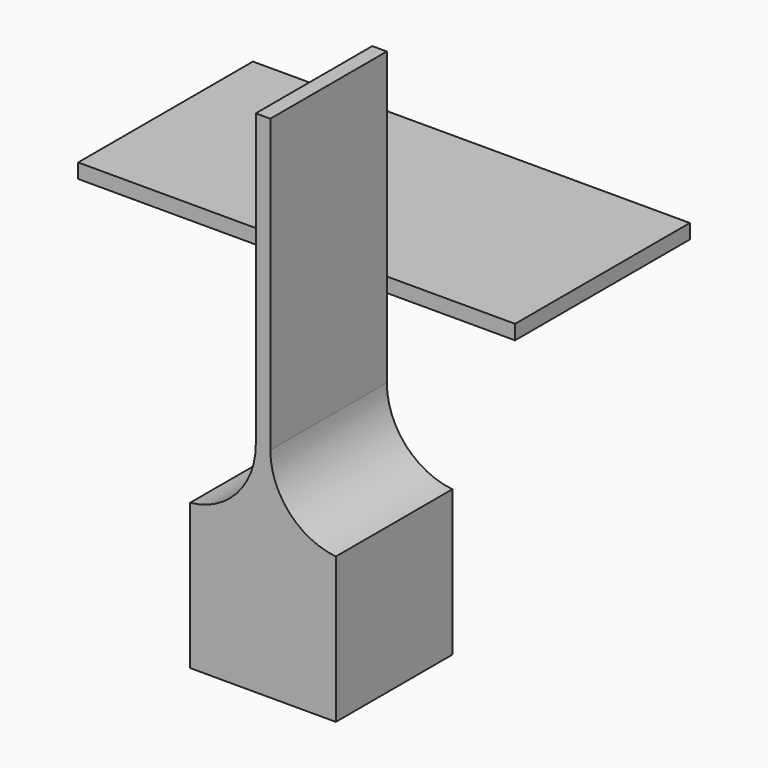
from build123d import *

# Parameters (mm, degrees)
F0_W        = 30
F0_H        = 15
F1_DEPTH    = 1
F2_W        = 10
F2_H        = 10
F3_DEPTH    = 10
F4_W        = 0.5
F4_H        = 10
F5_DEPTH    = 25
F6_T1_DEPTH = 10


# Not quite as in the source:
# - a fillet or chamfer that OpenCascade refuses, or shapes differently, is made with other operations: its cross-section is extruded or revolved along the edge and cut away or added


with BuildPart() as f1:
    # F0 (on Top) → F1 (new body)
    with BuildSketch(Plane.XY):
        with Locations((-29.4897666946, 42.1969963853)):
            Rectangle(F0_W, F0_H)
    extrude(amount=F1_DEPTH)


with BuildPart() as f3:
    # F2 (on Top) → F3 (new body)
    with BuildSketch(Plane.XY):
        with Locations((0.6839325652, -0.9021522023)):
            Rectangle(F2_W, F2_H)
    extrude(amount=F3_DEPTH)

    # F4 (on face) → F5 (join)
    with BuildSketch(Plane.XY.offset(10)):
        with Locations((0.4339325652, -0.9021522023)):
            Rectangle(F4_W, F4_H)
        with Locations((0.9339325652, -0.9021522023)):
            Rectangle(F4_W, F4_H)
    extrude(amount=F5_DEPTH)

    # F6: fillet of radius 5 on 2 edges, made by hand

    # F6_s2 → F6_t1 (join)
    with BuildSketch(Plane.XZ.offset(-4.0978477977)):
        with BuildLine():
            ThreePointArc((-4.3160674348, 10), (-1.1079681913, 11.6208352193), (0.1839325652, 14.9749371855))
            Line((0.1839325652, 14.9749371855), (0.1839325652, 10))
            Line((0.1839325652, 10), (-4.3160674348, 10))
        make_face()
        with BuildLine():
            ThreePointArc((5.6839325652, 10), (2.4758333216, 11.6208352193), (1.1839325652, 14.9749371855))
            Line((1.1839325652, 14.9749371855), (1.1839325652, 10))
            Line((1.1839325652, 10), (5.6839325652, 10))
        make_face()
    extrude(amount=F6_T1_DEPTH)


solid = Compound([f1.part, f3.part])
